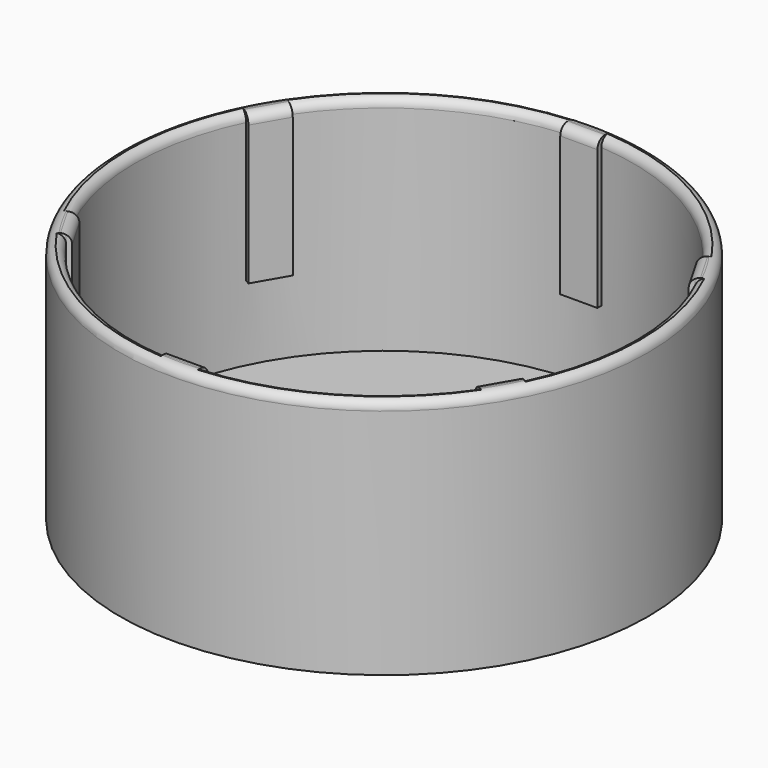
from build123d import *

# Parameters (mm, degrees)
F0_R         = 7.1
F1_DEPTH     = 0.5
F2_R         = 7.1
F2_R_2       = 6.7
F3_DEPTH     = 6
F4_W         = 1
F4_H         = 0.3
F5_DEPTH     = 4
F6_R         = 0.25
F7_T4_ANGLE  = 62.1313472273
F7_T10_ANGLE = 62.1313472273
F7_T16_ANGLE = 62.1313472273
F7_T22_ANGLE = 62.1313472273
F7_T28_ANGLE = 31.0651476548
F7_T33_ANGLE = 62.1313472273
F7_T39_ANGLE = 31.0651476548
F8_R         = 0.25


# Not quite as in the source:
# - a fillet or chamfer that OpenCascade refuses, or shapes differently, is made with other operations: its cross-section is extruded or revolved along the edge and cut away or added


with BuildPart() as f1:
    # F0 (on Top) → F1 (new body)
    with BuildSketch(Plane.XY):
        Circle(F0_R)
    extrude(amount=F1_DEPTH)

    # F2 (on face) → F3 (join)
    with BuildSketch(Plane.XY.offset(0.5)):
        Circle(F2_R)
        Circle(F2_R_2, mode=Mode.SUBTRACT)
    extrude(amount=F3_DEPTH)

    # F4 (on face) → F5 (join)
    with BuildSketch(Plane.XY.offset(6.5)):
        with Locations((0, 6.7)):
            Rectangle(F4_W, F4_H)
        Polygon((-5.9224663948, 2.8419872981), (-5.4224663948, 3.7080127019), (-5.6822740159, 3.8580127019), (-6.1822740159, 2.9919872981), align=None)
        Polygon((-5.4224663948, -3.7080127019), (-5.9224663948, -2.8419872981), (-6.1822740159, -2.9919872981), (-5.6822740159, -3.8580127019), align=None)
        with Locations((0, -6.7)):
            Rectangle(F4_W, F4_H)
        Polygon((5.9224663948, -2.8419872981), (5.4224663948, -3.7080127019), (5.6822740159, -3.8580127019), (6.1822740159, -2.9919872981), align=None)
        Polygon((5.4224663948, 3.7080127019), (5.9224663948, 2.8419872981), (6.1822740159, 2.9919872981), (5.6822740159, 3.8580127019), align=None)
    extrude(amount=-F5_DEPTH)

    # F6
    f6_edges = [f1.edges().sort_by_distance(p)[0] for p in [
        (-7.1, 0, 6.5),
    ]]
    fillet(f6_edges, radius=F6_R)

    # F7: fillet of radius 0.25 on 6 edges, made by hand


with BuildPart() as f7_tool2:
    # F7_s3 → F7_t4 (revolve)
    with BuildSketch(Plane(origin=(0, 0, 0), x_dir=(0, 0, 1), z_dir=(-0.4838067947, 0.8751748313, 0))):
        with BuildLine():
            ThreePointArc((6.5, -6.95), (6.4267766953, -6.7732233047), (6.25, -6.7))
            Line((6.25, -6.7), (6.5, -6.7))
            Line((6.5, -6.7), (6.5, -6.95))
        make_face()
    revolve(axis=Axis((0, 0, 6.5), (0, 0, 1)), revolution_arc=F7_T4_ANGLE)

    split(bisect_by=Plane.YZ.offset(-0.5), keep=Keep.BOTTOM)

    split(bisect_by=Plane(origin=(0.25, -0.4330127019, 0), x_dir=(0, 0, 1), z_dir=(0.5, -0.8660254038, 0)), keep=Keep.TOP)


with BuildPart() as f1_1:
    add(f1.part)

    # F7_t1: cut F7_tool2
    add(f7_tool2.part, mode=Mode.SUBTRACT)


with BuildPart() as f7_tool8:
    # F7_s9 → F7_t10 (revolve)
    with BuildSketch(Plane(origin=(0, 0, 0), x_dir=(0, 0, 1), z_dir=(0.5160202393, 0.8565763904, 0))):
        with BuildLine():
            ThreePointArc((6.5, -6.95), (6.4267766953, -6.7732233047), (6.25, -6.7))
            Line((6.25, -6.7), (6.5, -6.7))
            Line((6.5, -6.7), (6.5, -6.95))
        make_face()
    revolve(axis=Axis((0, 0, 6.5), (0, 0, 1)), revolution_arc=F7_T10_ANGLE)

    split(bisect_by=Plane(origin=(-0.25, 0.4330127019, 0), x_dir=(0, 0, 1), z_dir=(-0.5, 0.8660254038, 0)), keep=Keep.TOP)

    split(bisect_by=Plane(origin=(-0.25, -0.4330127019, 0), x_dir=(0, 0, 1), z_dir=(-0.5, -0.8660254038, 0)), keep=Keep.TOP)


with BuildPart() as f1_2:
    add(f1_1.part)

    # F7_t7: cut F7_tool8
    add(f7_tool8.part, mode=Mode.SUBTRACT)


with BuildPart() as f7_tool14:
    # F7_s15 → F7_t16 (revolve)
    with BuildSketch(Plane(origin=(0, 0, 0), x_dir=(0, 0, 1), z_dir=(0.999827034, -0.0185984409, 0))):
        with BuildLine():
            ThreePointArc((6.5, -6.95), (6.4267766953, -6.7732233047), (6.25, -6.7))
            Line((6.25, -6.7), (6.5, -6.7))
            Line((6.5, -6.7), (6.5, -6.95))
        make_face()
    revolve(axis=Axis((0, 0, 6.5), (0, 0, 1)), revolution_arc=F7_T16_ANGLE)

    split(bisect_by=Plane(origin=(0.25, 0.4330127019, 0), x_dir=(0, 0, 1), z_dir=(0.5, 0.8660254038, 0)), keep=Keep.TOP)

    split(bisect_by=Plane.YZ.offset(-0.5), keep=Keep.BOTTOM)


with BuildPart() as f1_3:
    add(f1_2.part)

    # F7_t13: cut F7_tool14
    add(f7_tool14.part, mode=Mode.SUBTRACT)


with BuildPart() as f7_tool20:
    # F7_s21 → F7_t22 (revolve)
    with BuildSketch(Plane(origin=(0, 0, 0), x_dir=(0, 0, 1), z_dir=(0.4838067947, -0.8751748313, 0))):
        with BuildLine():
            ThreePointArc((6.5, -6.95), (6.4267766953, -6.7732233047), (6.25, -6.7))
            Line((6.25, -6.7), (6.5, -6.7))
            Line((6.5, -6.7), (6.5, -6.95))
        make_face()
    revolve(axis=Axis((0, 0, 6.5), (0, 0, 1)), revolution_arc=F7_T22_ANGLE)

    split(bisect_by=Plane.YZ.offset(0.5), keep=Keep.TOP)

    split(bisect_by=Plane(origin=(-0.25, 0.4330127019, 0), x_dir=(0, 0, 1), z_dir=(-0.5, 0.8660254038, 0)), keep=Keep.TOP)


with BuildPart() as f1_4:
    add(f1_3.part)

    # F7_t19: cut F7_tool20
    add(f7_tool20.part, mode=Mode.SUBTRACT)


with BuildPart() as f7_tool26:
    # F7_s27 → F7_t28 (revolve)
    with BuildSketch(Plane(origin=(0, 0, 0), x_dir=(0, 0, 1), z_dir=(-0.5160123762, -0.8565811273, 0))):
        with BuildLine():
            ThreePointArc((6.5, -6.95), (6.4267766953, -6.7732233047), (6.25, -6.7))
            Line((6.25, -6.7), (6.5, -6.7))
            Line((6.5, -6.7), (6.5, -6.95))
        make_face()
    revolve(axis=Axis((0, 0, 6.5), (0, 0, 1)), revolution_arc=F7_T28_ANGLE)

    split(bisect_by=Plane(origin=(0.25, 0.4330127019, 0), x_dir=(0, 0, 1), z_dir=(0.5, 0.8660254038, 0)), keep=Keep.TOP)


with BuildPart() as f1_5:
    add(f1_4.part)

    # F7_t25: cut F7_tool26
    add(f7_tool26.part, mode=Mode.SUBTRACT)


with BuildPart() as f7_tool31:
    # F7_s32 → F7_t33 (revolve)
    with BuildSketch(Plane(origin=(0, 0, 0), x_dir=(0, 0, 1), z_dir=(-0.999827034, 0.0185984409, 0))):
        with BuildLine():
            ThreePointArc((6.5, -6.95), (6.4267766953, -6.7732233047), (6.25, -6.7))
            Line((6.25, -6.7), (6.5, -6.7))
            Line((6.5, -6.7), (6.5, -6.95))
        make_face()
    revolve(axis=Axis((0, 0, 6.5), (0, 0, 1)), revolution_arc=F7_T33_ANGLE)

    split(bisect_by=Plane(origin=(-0.25, -0.4330127019, 0), x_dir=(0, 0, 1), z_dir=(-0.5, -0.8660254038, 0)), keep=Keep.TOP)

    split(bisect_by=Plane.YZ.offset(0.5), keep=Keep.TOP)


with BuildPart() as f1_6:
    add(f1_5.part)

    # F7_t30: cut F7_tool31
    add(f7_tool31.part, mode=Mode.SUBTRACT)


with BuildPart() as f7_tool37:
    # F7_s38 → F7_t39 (revolve)
    with BuildSketch(Plane.XZ):
        with BuildLine():
            ThreePointArc((6.95, 6.5), (6.7732233047, 6.4267766953), (6.7, 6.25))
            Line((6.7, 6.25), (6.7, 6.5))
            Line((6.7, 6.5), (6.95, 6.5))
        make_face()
    revolve(axis=Axis((0, 0, 6.5), (0, 0, 1)), revolution_arc=F7_T39_ANGLE)

    split(bisect_by=Plane(origin=(0.25, -0.4330127019, 0), x_dir=(0, 0, 1), z_dir=(0.5, -0.8660254038, 0)), keep=Keep.TOP)


with BuildPart() as f1_7:
    add(f1_6.part)

    # F7_t36: cut F7_tool37
    add(f7_tool37.part, mode=Mode.SUBTRACT)

    # F8
    f8_edges = [f1_7.edges().sort_by_distance(p)[0] for p in [
        (-5.672466, 3.275, 6.5),
        (0, 6.55, 6.5),
        (5.672466, 3.275, 6.5),
        (5.672466, -3.275, 6.5),
        (0, -6.55, 6.5),
        (-5.672466, -3.275, 6.5),
    ]]
    fillet(f8_edges, radius=F8_R)


solid = f1_7.part
